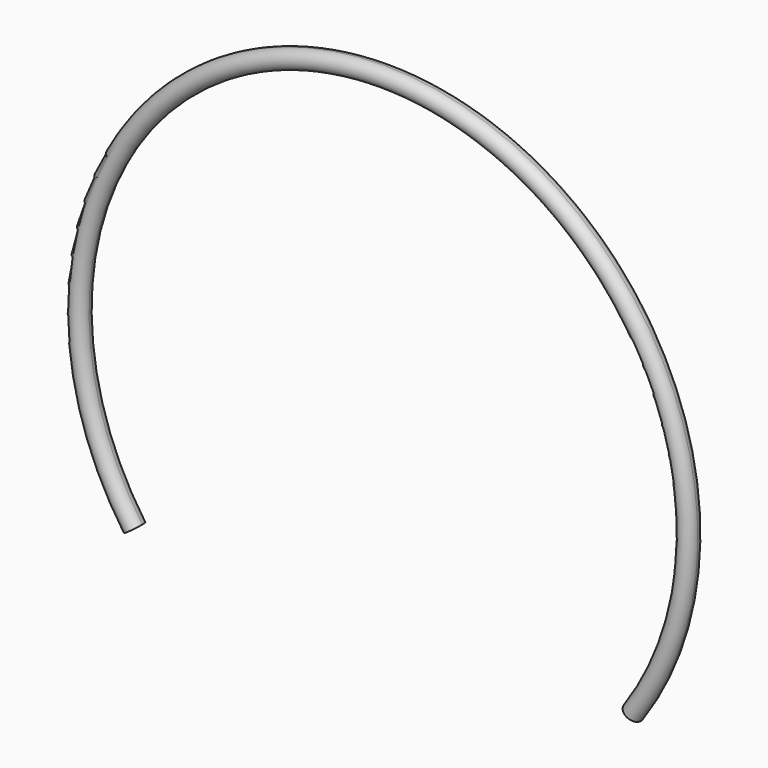
from build123d import *

# Parameters (mm, degrees)
F1_ANGLE_BACK = 35
F1_ANGLE      = 250


# Not quite as in the source:
# - a feature names something its author has since deleted; it is built from what else it names


with BuildPart() as f1:
    # F0 (on Top) → F1 (revolve)
    with BuildSketch(Plane.XY, mode=Mode.PRIVATE) as f1_sk:
        with BuildLine():
            ThreePointArc((-115.0866788832, 0), (-95.081537962, -20.0051409212), (-75.0763970407, 0))
            ThreePointArc((-75.0763970407, 0), (-95.081537962, 20.0051409212), (-115.0866788832, 0))
        make_face()
    revolve(f1_sk.sketch.rotate(Axis((-745.7624254748, 0, 0), (0, -1, 0)), -F1_ANGLE_BACK), axis=Axis((-745.7624254748, 0, 0), (0, -1, 0)), revolution_arc=F1_ANGLE)


solid = f1.part
